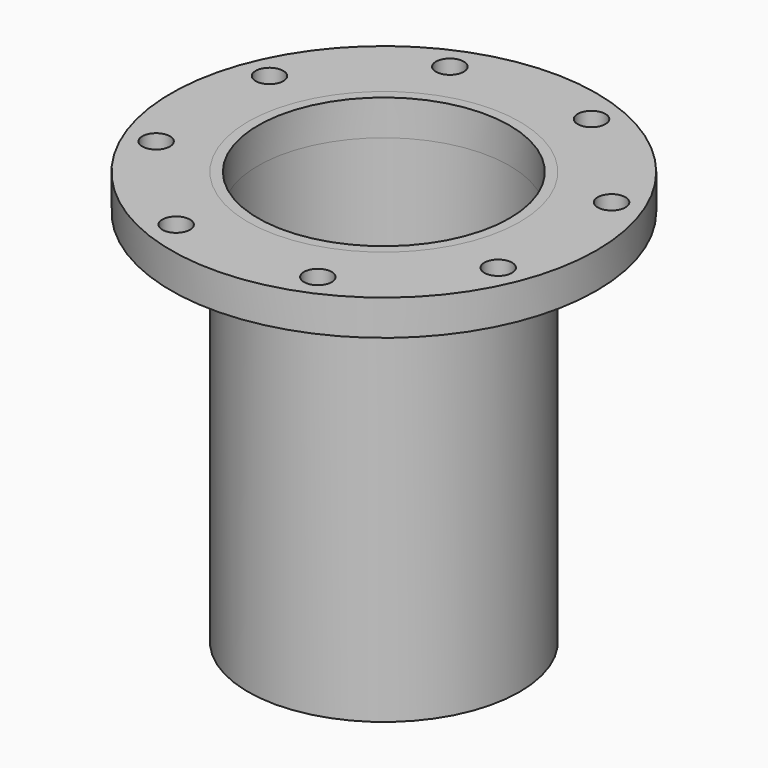
from build123d import *

# Parameters (mm, degrees)
F0_R     = 109.5375
F0_R_2   = 101.3587
F1_DEPTH = 304.8
F2_R     = 171.45
F2_R_2   = 11.176
F2_R_3   = 109.5375
F3_DEPTH = 28.575
F4_DEPTH = 28.575


# Not quite as in the source:
# - a feature names something its author has since deleted; it is built from what else it names


with BuildPart() as f1:
    # F0 (on Top) → F1 (new body)
    with BuildSketch(Plane.XY):
        Circle(F0_R)
        Circle(F0_R_2, mode=Mode.SUBTRACT)
    extrude(amount=F1_DEPTH)


with BuildPart() as f3:
    # F2 (on face) → F3 (new body)
    with BuildSketch(Plane.XY.offset(304.8)):
        Circle(F2_R)
        with Locations((-57.1059351947, -137.865923239)):
            Circle(F2_R_2, mode=Mode.SUBTRACT)
        with Locations((-137.865923239, -57.1059351947)):
            Circle(F2_R_2, mode=Mode.SUBTRACT)
        with Locations((57.1059351947, -137.865923239)):
            Circle(F2_R_2, mode=Mode.SUBTRACT)
        with Locations((137.865923239, -57.1059351947)):
            Circle(F2_R_2, mode=Mode.SUBTRACT)
        with Locations((-137.865923239, 57.1059351947)):
            Circle(F2_R_2, mode=Mode.SUBTRACT)
        with Locations((-57.1059351947, 137.865923239)):
            Circle(F2_R_2, mode=Mode.SUBTRACT)
        Circle(F2_R_3, mode=Mode.SUBTRACT)
        with Locations((137.865923239, 57.1059351947)):
            Circle(F2_R_2, mode=Mode.SUBTRACT)
        with Locations((57.1059351947, 137.865923239)):
            Circle(F2_R_2, mode=Mode.SUBTRACT)
    extrude(amount=F3_DEPTH)


with BuildPart() as f4:
    # F4 (new): a face of the model
    f4_faces = [f1.part.faces().sort_by_distance(p)[0] for p in [
        (-106.4393116382, 0, 304.8),
    ]]
    extrude(f4_faces, amount=F4_DEPTH)


solid = Compound([f1.part, f3.part, f4.part])
